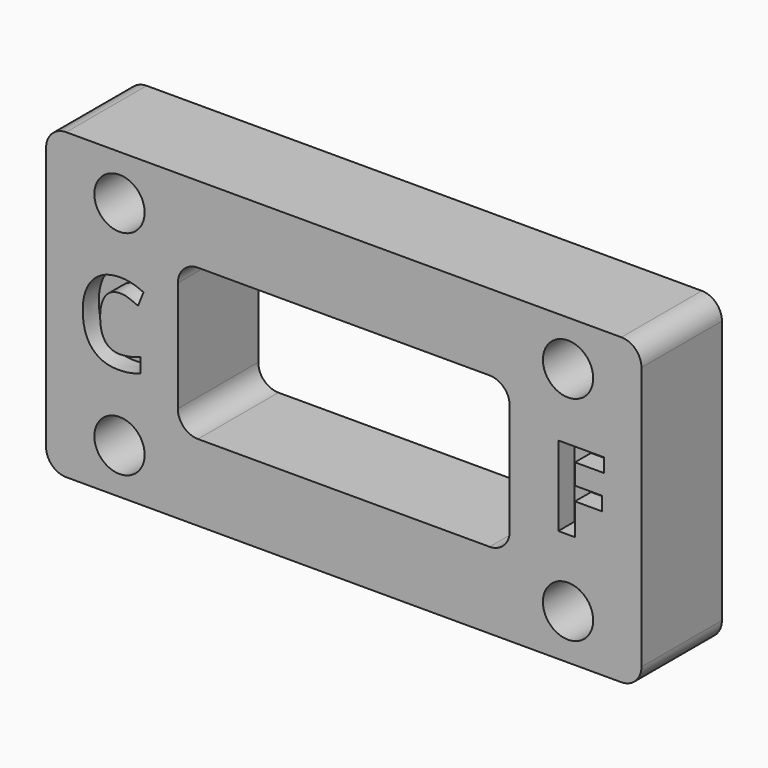
from build123d import *

# Parameters (mm, degrees)
F0_W         = 75.184
F0_H         = 38.354
F0_R         = 3.175
F0_W_2       = 41.91
F0_H_2       = 19.05
F1_DEPTH     = 12.7
F2_R         = 2.54
F3_TEXT_SIZE = 14.1111111111
F4_DEPTH     = 2.54


# Not quite as in the source:
# - Text() gives the source's letters only with a copy of the font that has no kerning and outlines rounded to 1/6400 em; it was checked with that copy


with BuildPart() as f1:
    # F0 (on Front) → F1 (new body)
    with BuildSketch(Plane.XZ):
        with Locations((37.592, 19.177)):
            Rectangle(F0_W, F0_H)
        with Locations((9.271, 5.715)):
            Circle(F0_R, mode=Mode.SUBTRACT)
        with Locations((65.913, 5.715)):
            Circle(F0_R, mode=Mode.SUBTRACT)
        with Locations((9.271, 32.639)):
            Circle(F0_R, mode=Mode.SUBTRACT)
        with Locations((37.592, 19.177)):
            Rectangle(F0_W_2, F0_H_2, mode=Mode.SUBTRACT)
        with Locations((65.913, 32.639)):
            Circle(F0_R, mode=Mode.SUBTRACT)
    extrude(amount=F1_DEPTH)

    # F2
    f2_edges = [f1.edges().sort_by_distance(p)[0] for p in [
        (0, -6.35, 38.354),
        (0, -6.35, 0),
        (75.184, -6.35, 38.354),
        (75.184, -6.35, 0),
        (16.637, -6.35, 28.702),
        (58.547, -6.35, 9.652),
        (58.547, -6.35, 28.702),
        (16.637, -6.35, 9.652),
    ]]
    fillet(f2_edges, radius=F2_R)

    # F3 (on face) → F4 (cut)
    with BuildSketch(Plane.XZ.offset(12.7)):
        with Locations((3.81, 14.224)):
            Text('C', F3_TEXT_SIZE, font='Open Sans', font_style=FontStyle.BOLD, text_align=(TextAlign.LEFT, TextAlign.BOTTOM))
        with Locations((63.41665625, 14.224)):
            Text('F', F3_TEXT_SIZE, font='Open Sans', font_style=FontStyle.BOLD, text_align=(TextAlign.LEFT, TextAlign.BOTTOM))
    extrude(amount=-F4_DEPTH, mode=Mode.SUBTRACT)


solid = f1.part
